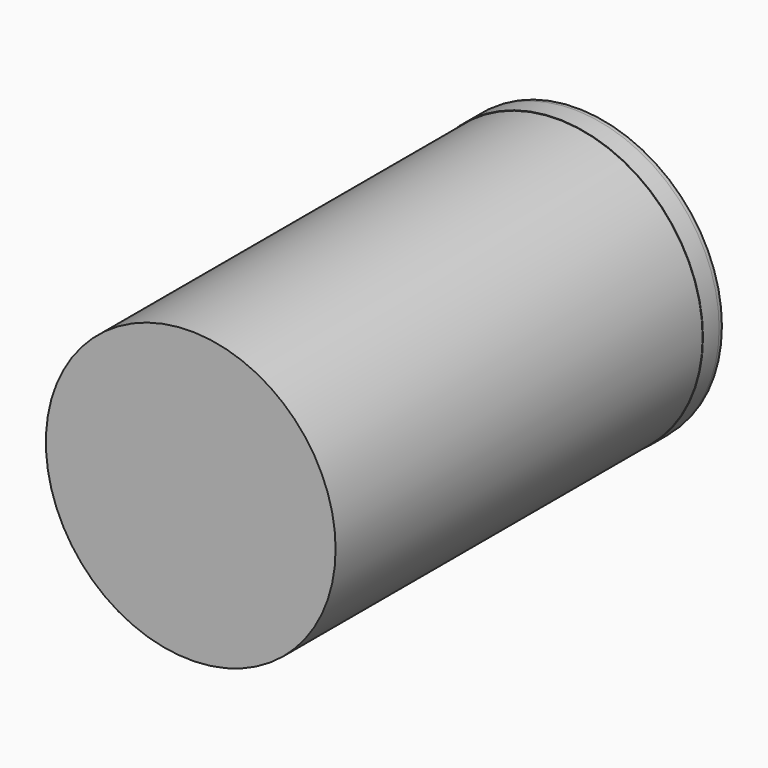
from build123d import *

# Parameters (mm, degrees)
F0_R     = 38.2126464565
F0_R_2   = 38.1
F1_DEPTH = 6.35
F2_DEPTH = 127


# Not quite as in the source:
# - a fillet or chamfer that OpenCascade refuses, or shapes differently, is made with other operations: its cross-section is extruded or revolved along the edge and cut away or added
# - the program builds the solid bodies; features that only make, move or delete a surface that nothing else refers to are left out


with BuildPart() as f1:
    # F0 (on Front) → F1 (new body)
    with BuildSketch(Plane.XZ):
        Circle(F0_R)
        Circle(F0_R_2, mode=Mode.SUBTRACT)
    extrude(amount=F1_DEPTH)

    # F4: fillet of radius 5.08 on 1 edges, made by hand

    # F4_s1 → F4_t2 (revolve, cut)
    with BuildSketch(Plane.XY):
        with BuildLine():
            ThreePointArc((38.2126464565, -1.0638603171), (38.1844063479, -0.5289565878), (38.1, 0))
            Line((38.1, 0), (38.1993470709, 0.0212772063))
            ThreePointArc((38.1993470709, 0.0212772063), (38.1563232283, 0.1016), (38.2126464565, 0.1016))
            Line((38.2126464565, 0.1016), (38.3142464565, 0))
            Line((38.3142464565, 0), (38.3142464565, -1.0638603171))
            Line((38.3142464565, -1.0638603171), (38.2126464565, -1.0638603171))
        make_face()
    revolve(axis=Axis((0, 0, 0), (0, -1, 0)), mode=Mode.SUBTRACT)


with BuildPart() as f2:
    # F0 (on Front) → F2 (new body)
    with BuildSketch(Plane.XZ):
        Circle(F0_R_2)
    extrude(amount=F2_DEPTH)


solid = Compound([f1.part, f2.part])
